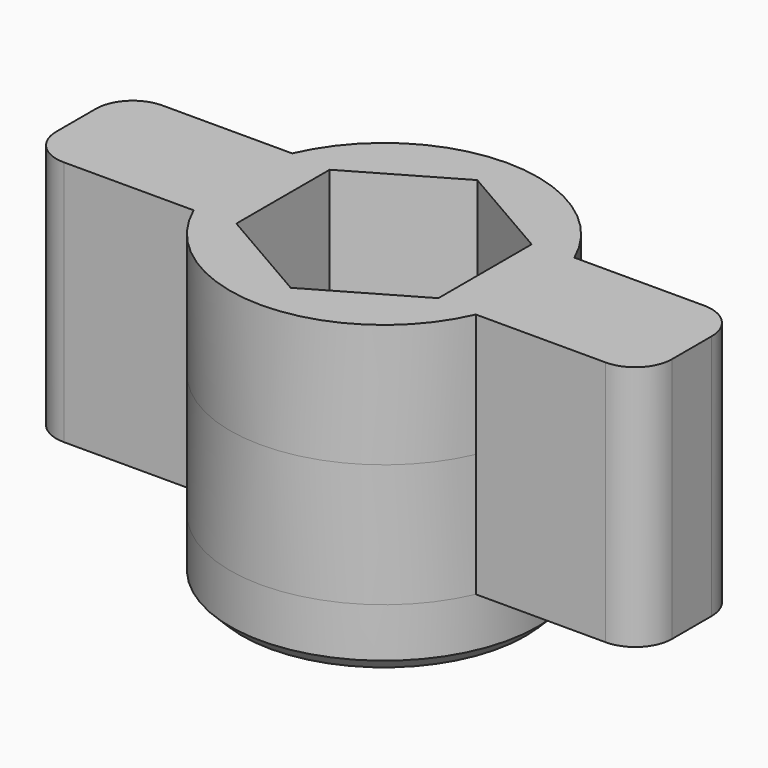
from build123d import *

# Parameters (mm, degrees)
F0_R     = 6.25
F0_R_2   = 2.6
F1_DEPTH = 7.5
F3_DEPTH = 5
F4_SIZE  = 0.5
F5_R     = 2.6
F6_DEPTH = 4


# Not quite as in the source:
# - a feature names something its author has since deleted; it is built from what else it names


with BuildPart() as f1:
    # F0 (on Top) → F1 (new body)
    with BuildSketch(Plane.XY):
        Circle(F0_R)
        Circle(F0_R_2, mode=Mode.SUBTRACT)
    extrude(amount=F1_DEPTH)

    # F2 (on face) → F3 (join, symmetric)
    with BuildSketch(Plane.XY.offset(7.5)):
        with BuildLine():
            Line((11, 2.5), (5.7282196187, 2.5))
            ThreePointArc((5.7282196187, 2.5), (6.1181644558, 1.2769352731), (6.25, 0))
            ThreePointArc((6.25, 0), (6.1181644558, -1.2769352731), (5.7282196187, -2.5))
            Line((5.7282196187, -2.5), (11, -2.5))
            ThreePointArc((11, -2.5), (12.0606601718, -2.0606601718), (12.5, -1))
            Line((12.5, -1), (12.5, 1))
            ThreePointArc((12.5, 1), (12.0606601718, 2.0606601718), (11, 2.5))
        make_face()
        with BuildLine():
            ThreePointArc((-5.7282196187, -2.5), (-6.25, 0), (-5.7282196187, 2.5))
            Line((-5.7282196187, 2.5), (-11, 2.5))
            ThreePointArc((-11, 2.5), (-12.0606601718, 2.0606601718), (-12.5, 1))
            Line((-12.5, 1), (-12.5, -1))
            ThreePointArc((-12.5, -1), (-12.0606601718, -2.0606601718), (-11, -2.5))
            Line((-11, -2.5), (-5.7282196187, -2.5))
        make_face()
        with BuildLine():
            ThreePointArc((6.25, 0), (6.1181644558, 1.2769352731), (5.7282196187, 2.5))
            ThreePointArc((5.7282196187, 2.5), (0, 6.25), (-5.7282196187, 2.5))
            ThreePointArc((-5.7282196187, 2.5), (-6.25, 0), (-5.7282196187, -2.5))
            ThreePointArc((-5.7282196187, -2.5), (0, -6.25), (5.7282196187, -2.5))
            ThreePointArc((5.7282196187, -2.5), (6.1181644558, -1.2769352731), (6.25, 0))
        make_face()
        Polygon((-4.1, 2.3671361037), (0, 4.7342722074), (4.1, 2.3671361037), (4.1, -2.3671361037), (0, -4.7342722074), (-4.1, -2.3671361037), align=None, mode=Mode.SUBTRACT)
    extrude(amount=F3_DEPTH, both=True)

    # F4
    f4_edges = [f1.edges().sort_by_distance(p)[0] for p in [
        (-6.25, 0, 0),
        (-2.6, 0, 0),
    ]]
    chamfer(f4_edges, length=F4_SIZE)

    # F5 (on face) → F6 (cut)
    with BuildSketch(Plane.XY.offset(7.5)):
        Polygon((4.1, -2.3671361037), (4.1, 2.3671361037), (0, 4.7342722074), (-4.1, 2.3671361037), (-4.1, -2.3671361037), (0, -4.7342722074), align=None)
        Circle(F5_R, mode=Mode.SUBTRACT)
    extrude(amount=-F6_DEPTH, mode=Mode.SUBTRACT)


solid = f1.part
